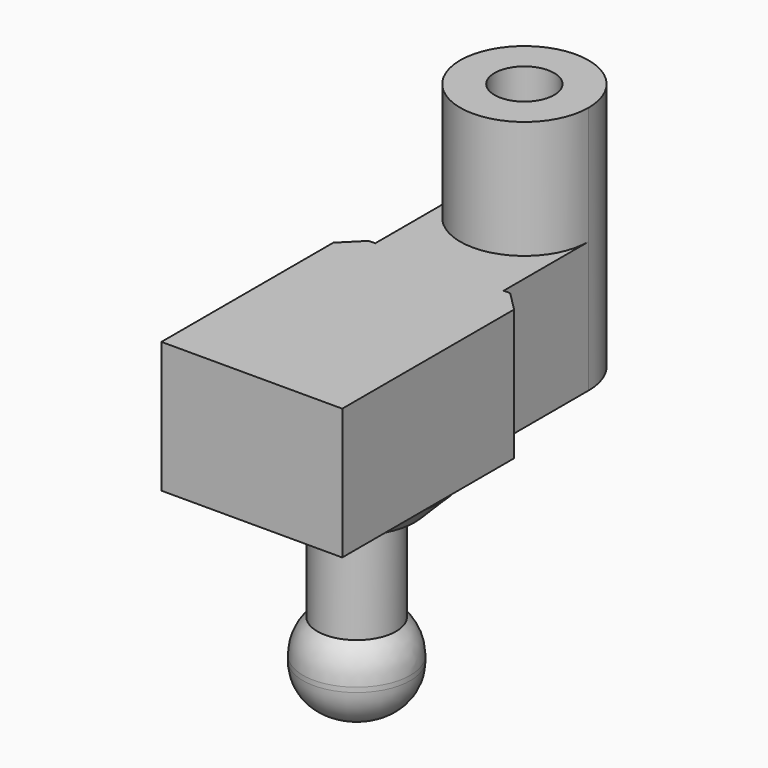
from build123d import *

# Parameters (mm, degrees)
F0_R         = 2.8766712164
F1_DEPTH     = 19
F0_R_2       = 3
F2_DEPTH     = 16.5
F3_START     = -10.3
F0_R_3       = 4.1
F3_DEPTH     = 6.2
F0_R_4       = 6.4405757452
F4_DEPTH     = 2.5
F5_DEPTH     = 10
F6_R         = 3.25
F8_SIZE      = 2
F9_START     = 9
F0_R_5       = 2.2754716525
F9_DEPTH     = 10
F10_S5_R     = 2.8766712164
F10_T6_DEPTH = 7
F11_SIZE     = 1.5


# Not quite as in the source:
# - a fillet or chamfer that OpenCascade refuses, or shapes differently, is made with other operations: its cross-section is extruded or revolved along the edge and cut away or added


with BuildPart() as f1:
    # F0 (on Top) → F1 (new body)
    with BuildSketch(Plane.XY):
        with BuildLine():
            Line((2, 26.0571271565), (2, 25.9428728435))
            ThreePointArc((2, 25.9428728435), (6.9283975578, 21.0999167478), (11.8, 26))
            ThreePointArc((11.8, 26), (10.4404727363, 29.3875515556), (7.1162793435, 30.8953838438))
            Line((7.1162793435, 30.8953838438), (6.7435880271, 30.8953838438))
            ThreePointArc((6.7435880271, 30.8953838438), (6.7074201677, 30.8952459595), (6.6712544109, 30.8948323144))
            ThreePointArc((6.6712544109, 30.8948323144), (3.3747800634, 29.4037670445), (2, 26.0571271565))
        make_face()
        with Locations((6.8998334943, 26)):
            Circle(F0_R, mode=Mode.SUBTRACT)
    extrude(amount=F1_DEPTH)

    # F0 (on Top) → F9 (join)
    with BuildSketch(Plane.XY.offset(F9_START)):
        with Locations((6.8998334943, 26)):
            Circle(F0_R)
        with Locations((6.8998334943, 26)):
            Circle(F0_R_5, mode=Mode.SUBTRACT)
    extrude(amount=F9_DEPTH)

    # F10: chamfer of 1.25 on 1 edges, made by hand


with BuildPart() as f2:
    # F0 (on Top) → F2 (new body)
    with BuildSketch(Plane.XY):
        with Locations((6.9, 10)):
            Circle(F0_R_2)
    extrude(amount=-F2_DEPTH)

    # F0 (on Top) → F3 (join)
    with BuildSketch(Plane.XY.offset(F3_START)):
        with Locations((6.9, 10)):
            Circle(F0_R_3)
        with Locations((6.9, 10)):
            Circle(F0_R_2, mode=Mode.SUBTRACT)
    extrude(amount=-F3_DEPTH)

    # F0 (on Top) → F4 (join)
    with BuildSketch(Plane.XY):
        with Locations((6.9, 10)):
            Circle(F0_R_4)
        with Locations((6.9, 10)):
            Circle(F0_R_3, mode=Mode.SUBTRACT)
        with Locations((6.9, 10)):
            Circle(F0_R_3)
        with Locations((6.9, 10)):
            Circle(F0_R_2, mode=Mode.SUBTRACT)
    extrude(amount=-F4_DEPTH)

    # F6
    f6_edges = [f2.edges().sort_by_distance(p)[0] for p in [
        (2.8, 10, -16.5),
    ]]
    fillet(f6_edges, radius=F6_R)

    # F7: fillet of radius 3.6 on 1 edges, made by hand

    # F7_s1 → F7_t2 (revolve, cut)
    with BuildSketch(Plane.XZ.offset(-10)):
        with BuildLine():
            ThreePointArc((11, -12.8903667694), (10.7136083052, -11.4832420415), (9.9, -10.3))
            Line((9.9, -10.3), (11, -10.3))
            Line((11, -10.3), (11, -12.8903667694))
        make_face()
    revolve(axis=Axis((6.9, 10, -10.3), (0, 0, 1)), mode=Mode.SUBTRACT)

    # F8
    f8_edges = [f2.edges().sort_by_distance(p)[0] for p in [
        (0.459424, 10, -2.5),
    ]]
    chamfer(f8_edges, length=F8_SIZE)


with BuildPart() as f5:
    # F0 (on Top) → F5 (new body)
    with BuildSketch(Plane.XY):
        with BuildLine():
            Line((2, 25.9428728435), (2, 17.8943023658))
            Line((2, 17.8943023658), (11.8, 17.8943023658))
            Line((11.8, 17.8943023658), (11.8, 26))
            ThreePointArc((11.8, 26), (6.9283975578, 21.0999167478), (2, 25.9428728435))
        make_face()
        Polygon((0, 17.8943023658), (0, 0), (13.8, 0), (13.8, 17.8943023658), (11.8, 17.8943023658), (2, 17.8943023658), align=None)
        with Locations((6.9, 10)):
            Circle(F0_R_4, mode=Mode.SUBTRACT)
        with Locations((6.9, 10)):
            Circle(F0_R_4)
        with Locations((6.9, 10)):
            Circle(F0_R_3, mode=Mode.SUBTRACT)
        with Locations((6.9, 10)):
            Circle(F0_R_3)
        with Locations((6.9, 10)):
            Circle(F0_R_2, mode=Mode.SUBTRACT)
        with Locations((6.9, 10)):
            Circle(F0_R_2)
    extrude(amount=F5_DEPTH)

    # F11
    f11_edges = [f5.edges().sort_by_distance(p)[0] for p in [
        (0, 17.894302, 5),
        (13.8, 17.894302, 5),
    ]]
    chamfer(f11_edges, length=F11_SIZE)


with BuildPart() as f10_tool2:
    # F10_s3 → F10_t4 (revolve)
    with BuildSketch(Plane.XZ.offset(-26)):
        Polygon((10.4253051468, 9), (9.1753051468, 10.25), (9.1753051468, 9), align=None)
    revolve(axis=Axis((6.8998334943, 26, 9), (0, 0, 1)))

    # F10_s5 → F10_t6 (intersect, symmetric)
    with BuildSketch(Plane.XY.offset(9.6)):
        with Locations((6.8998334943, 26)):
            Circle(F10_S5_R)
    extrude(amount=F10_T6_DEPTH, both=True, mode=Mode.INTERSECT)


with BuildPart() as f1_1:
    add(f1.part)

    # F10_t1: cut F10_tool2
    add(f10_tool2.part, mode=Mode.SUBTRACT)


solid = Compound([f2.part, f5.part, f1_1.part])
